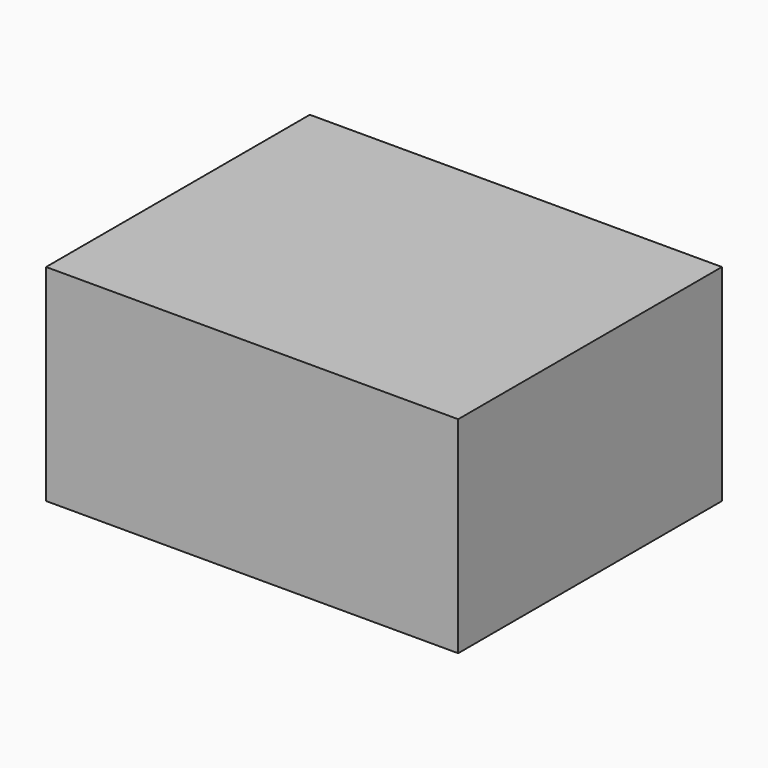
from build123d import *

# Parameters (mm, degrees)
F0_W     = 127
F0_H     = 63.5
F1_DEPTH = 101.6


# Not quite as in the source:
# - the program builds the solid bodies; features that only make, move or delete a surface that nothing else refers to are left out


with BuildPart() as f1:
    # F0 (on Front) → F1 (new body)
    with BuildSketch(Plane.XZ):
        with Locations((63.5, 31.75)):
            Rectangle(F0_W, F0_H)
    extrude(amount=F1_DEPTH)


solid = f1.part
